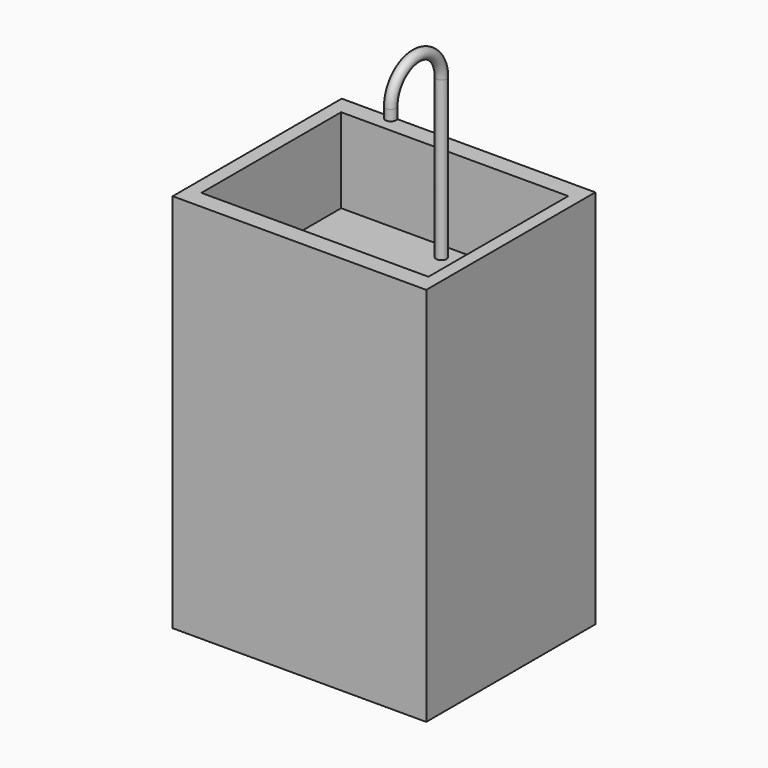
from build123d import *

# Parameters (mm, degrees)
F0_W     = 600
F0_H     = 500
F1_DEPTH = 900
F2_W     = 537.3239591718
F2_H     = 413.3979640901
F3_DEPTH = 200
F6_R     = 12.5


# Not quite as in the source:
# - a feature names something its author has since deleted; it is built from what else it names


with BuildPart() as f1:
    # F0 (on Top) → F1 (new body)
    with BuildSketch(Plane.XY):
        with Locations((300, 250)):
            Rectangle(F0_W, F0_H)
    extrude(amount=F1_DEPTH)

    # F2 (on face) → F3 (cut)
    with BuildSketch(Plane.XY.offset(900)):
        with Locations((301.7210625112, 250.2208668739)):
            Rectangle(F2_W, F2_H)
    extrude(amount=-F3_DEPTH, mode=Mode.SUBTRACT)

    # F7: sweep along a path in F5
    with BuildLine(Plane(origin=(300, 0, 0), x_dir=(0, -1, 0), z_dir=(-1, 0, 0))) as f7_path:
        Line((-420, 589.8187315079), (-420, 1075))
        ThreePointArc((-420, 1075), (-398.033008589, 1128.033008589), (-345, 1150))
        ThreePointArc((-345, 1150), (-291.966991411, 1128.033008589), (-270, 1075))
        Line((-270, 1075), (-270, 1050))
    # F6 (on face) → F7 (sweep)
    with BuildSketch(Plane.XY.offset(700)):
        with Locations((300.0000119209, 420.0000464916)):
            Circle(F6_R)
    sweep(path=f7_path.line)


solid = f1.part
